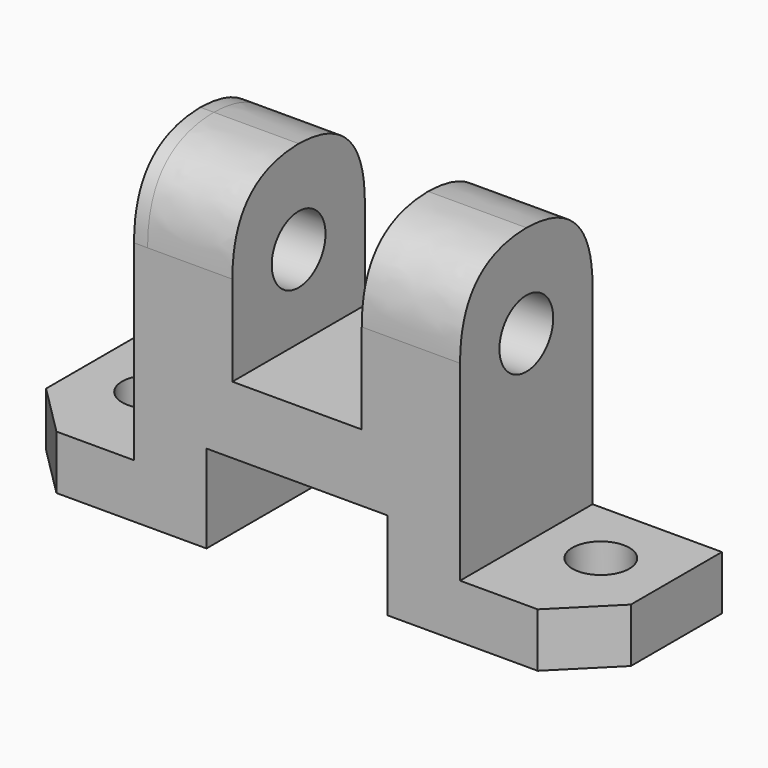
from build123d import *

# Parameters (mm, degrees)
F0_W         = 113
F0_H         = 32
F1_DEPTH     = 64
F2_W         = 25
F2_H         = 32
F3_DEPTH     = 53.5432
F4_W         = 35
F4_H         = 17
F5_DEPTH     = 34.544
F6_SIZE      = 10
F7_W         = 25
F7_H         = 34
F8_DEPTH     = 33.274
F9_R         = 5.5
F10_DEPTH    = 25.4
F11_R        = 6.5
F12_DEPTH    = 82.296
F13_T1_DEPTH = 101.7833830538
F13_T3_DEPTH = 101.7833830538


# Not quite as in the source:
# - a fillet or chamfer that OpenCascade refuses, or shapes differently, is made with other operations: its cross-section is extruded or revolved along the edge and cut away or added


with BuildPart() as f1:
    # F0 (on Top) → F1 (new body)
    with BuildSketch(Plane.XY):
        with Locations((-26.9756987691, -17.7779501617)):
            Rectangle(F0_W, F0_H)
    extrude(amount=F1_DEPTH)

    # F2 (on face) → F3 (cut)
    with BuildSketch(Plane.XY.offset(64)):
        with Locations((-70.9756987691, -17.7779501617)):
            Rectangle(F2_W, F2_H)
        with Locations((17.0243012309, -17.7779501617)):
            Rectangle(F2_W, F2_H)
    extrude(amount=-F3_DEPTH, mode=Mode.SUBTRACT)

    # F4 (on face) → F5 (cut)
    with BuildSketch(Plane.XZ.offset(33.7779501617)):
        with Locations((-26.9756987691, 8.5)):
            Rectangle(F4_W, F4_H)
    extrude(amount=-F5_DEPTH, mode=Mode.SUBTRACT)

    # F6
    f6_edges = [f1.edges().sort_by_distance(p)[0] for p in [
        (29.524301, -33.77795, 5.2284),
        (-83.475699, -33.77795, 5.2284),
    ]]
    chamfer(f6_edges, length=F6_SIZE)

    # F7 (on face) → F8 (cut)
    with BuildSketch(Plane.XZ.offset(33.7779501617)):
        with Locations((-26.9756987691, 47)):
            Rectangle(F7_W, F7_H)
    extrude(amount=-F8_DEPTH, mode=Mode.SUBTRACT)

    # F9 (on face) → F10 (cut)
    with BuildSketch(Plane.XY.offset(10.4568)):
        with Locations((-70.4708987691, -14.7827501617)):
            Circle(F9_R)
        with Locations((16.5243012309, -14.7779501617)):
            Circle(F9_R)
    extrude(amount=-F10_DEPTH, mode=Mode.SUBTRACT)

    # F11 (on face) → F12 (cut)
    with BuildSketch(Plane.YZ.offset(4.5243012309)):
        with Locations((-17.7779501617, 46)):
            Circle(F11_R)
    extrude(amount=-F12_DEPTH, mode=Mode.SUBTRACT)

    # F13: fillet of radius 16.5566766108 on 4 edges, made by hand

    # F13_s2 → F13_t1 (cut)
    with BuildSketch(Plane.YZ.offset(-55.867390296)):
        with BuildLine():
            add(Edge.make_bspline(
                [(-33.7779501617, 47.4433233892), (-33.7779501617, 64), (-17.2212735509, 64)],
                knots=[0, 0, 0, 1, 1, 1], degree=2, weights=[1, 1, 1]))
            Line((-17.2212735509, 64), (-33.7779501617, 64))
            Line((-33.7779501617, 64), (-33.7779501617, 47.4433233892))
        make_face()
        with BuildLine():
            add(Edge.make_bspline(
                [(-1.7779501617, 47.4433233892), (-1.7779501617, 64), (-18.3346267724, 64)],
                knots=[0, 0, 0, 1, 1, 1], degree=2, weights=[1, 1, 1]))
            Line((-18.3346267724, 64), (-1.7779501617, 64))
            Line((-1.7779501617, 64), (-1.7779501617, 47.4433233892))
        make_face()
    extrude(amount=F13_T1_DEPTH, mode=Mode.SUBTRACT)

    # F13_s4 → F13_t3 (cut)
    with BuildSketch(Plane.YZ.offset(-99.867390296)):
        with BuildLine():
            add(Edge.make_bspline(
                [(-33.7779501617, 47.4433233892), (-33.7779501617, 64), (-17.2212735509, 64)],
                knots=[0, 0, 0, 1, 1, 1], degree=2, weights=[1, 1, 1]))
            Line((-17.2212735509, 64), (-33.7779501617, 64))
            Line((-33.7779501617, 64), (-33.7779501617, 47.4433233892))
        make_face()
        with BuildLine():
            add(Edge.make_bspline(
                [(-1.7779501617, 47.4433233892), (-1.7779501617, 64), (-18.3346267724, 64)],
                knots=[0, 0, 0, 1, 1, 1], degree=2, weights=[1, 1, 1]))
            Line((-18.3346267724, 64), (-1.7779501617, 64))
            Line((-1.7779501617, 64), (-1.7779501617, 47.4433233892))
        make_face()
    extrude(amount=F13_T3_DEPTH, mode=Mode.SUBTRACT)


solid = f1.part
